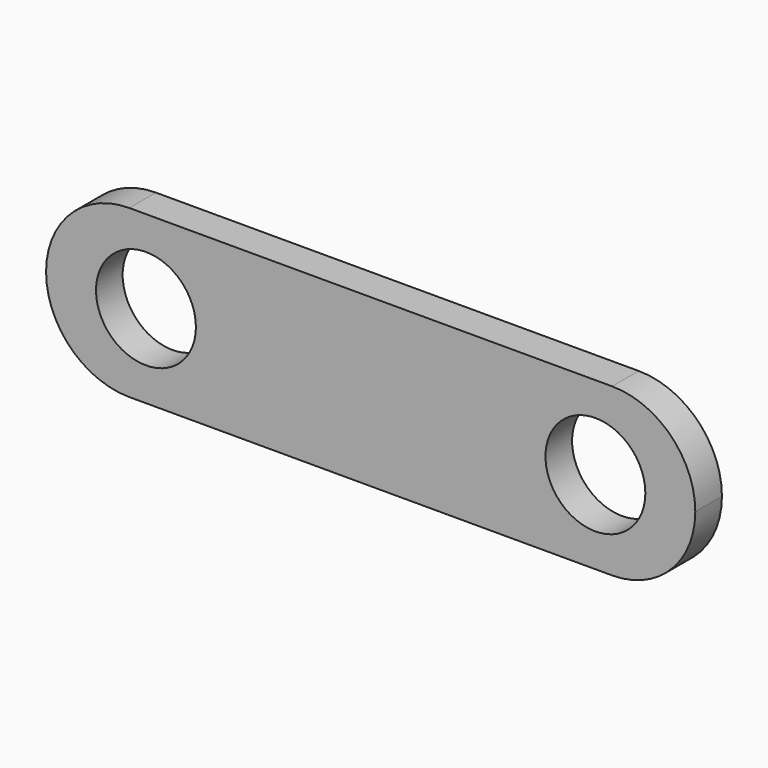
from build123d import *

# Parameters (mm, degrees)
F0_W     = 19.5
F0_H     = 5
F0_R     = 1.5
F1_DEPTH = 1
F2_R     = 2.49999


# Not quite as in the source:
# - a fillet or chamfer is up to 0.001 mm smaller than in the source, because OpenCascade refuses the exact size


with BuildPart() as f1:
    # F0 (on Front) → F1 (new body)
    with BuildSketch(Plane.XZ):
        with Locations((9.75, 2.5)):
            Rectangle(F0_W, F0_H)
        with Locations((3, 2.5)):
            Circle(F0_R, mode=Mode.SUBTRACT)
        with Locations((16.5, 2.5)):
            Circle(F0_R, mode=Mode.SUBTRACT)
    extrude(amount=F1_DEPTH)

    # F2 (radius 2.5 in the source; OpenCascade refuses exactly that, so slightly less here)
    f2_edges = [f1.edges().sort_by_distance(p)[0] for p in [
        (0, -0.5, 5),
        (0, -0.5, 0),
        (19.5, -0.5, 5),
        (19.5, -0.5, 0),
    ]]
    fillet(f2_edges, radius=F2_R)


solid = f1.part
